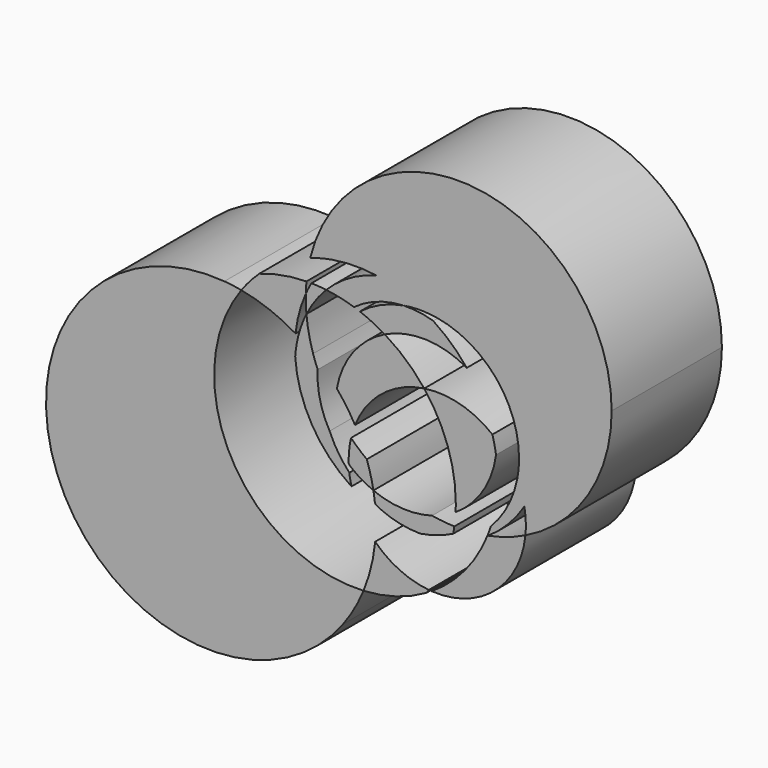
from build123d import *

# Parameters (mm, degrees)
F1_DEPTH = 25.4


with BuildPart() as f1:
    # F0 (on Front) → F1 (new body)
    with BuildSketch(Plane.XZ):
        with BuildLine():
            ThreePointArc((40.1538575824, -54.5525371766), (34.8112838881, -53.101159825), (30.2607130008, -49.9480828366))
            ThreePointArc((30.2607130008, -49.9480828366), (29.5067805021, -54.3549736685), (28.1146409687, -58.6036262239))
            ThreePointArc((28.1146409687, -58.6036262239), (34.1030907269, -57.5733618162), (39.691420026, -55.1872455363))
            ThreePointArc((39.691420026, -55.1872455363), (39.9249388458, -54.8715671271), (40.1538575824, -54.5525371766))
        make_face()
    extrude(amount=F1_DEPTH)


with BuildPart() as f1b:
    # F0 (on Front) → F1, piece 2 (new body)
    with BuildSketch(Plane.XZ):
        with BuildLine():
            ThreePointArc((24.3295831314, -65.2665911695), (26.4328949575, -62.0548490079), (28.1146409687, -58.6036262239))
            ThreePointArc((28.1146409687, -58.6036262239), (3.7618317001, -44.9945627843), (5.5896871945, -17.1570903547))
            ThreePointArc((5.5896871945, -17.1570903547), (4.0379815695, -16.9081548594), (2.4754848513, -16.7397409859))
            ThreePointArc((2.4754848513, -16.7397409859), (-6.670828805, -50.0432179604), (24.3295831314, -65.2665911695))
        make_face()
        with BuildLine():
            ThreePointArc((2.4754848513, -16.7397409859), (-27.7189775168, -59.5222653089), (24.3295831314, -65.2665911695))
            ThreePointArc((24.3295831314, -65.2665911695), (-6.670828805, -50.0432179604), (2.4754848513, -16.7397409859))
        make_face()
    extrude(amount=F1_DEPTH)


with BuildPart() as f1c:
    # F0 (on Front) → F1, piece 3 (new body)
    with BuildSketch(Plane.XZ):
        with BuildLine():
            ThreePointArc((15.5259313509, -24.7108479388), (18.6165177504, -34.7842088044), (25.8966178224, -42.4015880363))
            ThreePointArc((25.8966178224, -42.4015880363), (25.6616341127, -41.3572292778), (25.4955819125, -40.2997184139))
            ThreePointArc((25.4955819125, -40.2997184139), (23.4256571039, -37.6786317178), (21.8713846988, -34.7224650322))
            ThreePointArc((21.8713846988, -34.7224650322), (20.0913666116, -30.2566972991), (19.6726895469, -25.4675162258))
            ThreePointArc((19.6726895469, -25.4675162258), (19.221825797, -24.3258278708), (18.8210952423, -23.1655927897))
            ThreePointArc((18.8210952423, -23.1655927897), (17.4751466685, -22.1634611108), (16.075953424, -21.2371222257))
            ThreePointArc((16.075953424, -21.2371222257), (15.7246867633, -22.9619109348), (15.5259313509, -24.7108479388))
        make_face()
        with BuildLine():
            ThreePointArc((17.5902280452, -17.1382927375), (16.7211824063, -19.1463639854), (16.075953424, -21.2371222257))
            ThreePointArc((16.075953424, -21.2371222257), (17.4751466685, -22.1634611108), (18.8210952423, -23.1655927897))
            ThreePointArc((18.8210952423, -23.1655927897), (18.0407428379, -20.1856217155), (17.5902280452, -17.1382927375))
        make_face()
    extrude(amount=F1_DEPTH)


with BuildPart() as f1d:
    # F0 (on Front) → F1, piece 4 (new body)
    with BuildSketch(Plane.XZ):
        with BuildLine():
            ThreePointArc((8.9074729487, -13.4113681026), (7.1586729424, -15.2045936945), (5.5896871945, -17.1570903547))
            ThreePointArc((5.5896871945, -17.1570903547), (10.7582958294, -18.606057575), (15.5914806817, -20.94151158))
            ThreePointArc((15.5914806817, -20.94151158), (16.2501882549, -17.3285688299), (17.4789014653, -13.8677141914))
            ThreePointArc((17.4789014653, -13.8677141914), (17.5218559184, -12.8490388813), (17.6016231545, -11.8325834418))
            ThreePointArc((17.6016231545, -11.8325834418), (13.1897424114, -12.265100016), (8.9074729487, -13.4113681026))
        make_face()
    extrude(amount=F1_DEPTH)


with BuildPart() as f1e:
    # F0 (on Front) → F1, piece 5 (new body)
    with BuildSketch(Plane.XZ):
        with BuildLine():
            ThreePointArc((50.9276188863, -42.3062252748), (46.7662943353, -49.2544379076), (40.6765473403, -54.5938444613))
            ThreePointArc((40.6765473403, -54.5938444613), (52.276756188, -50.7389787125), (57.9506689588, -39.9116268146))
            ThreePointArc((57.9506689588, -39.9116268146), (54.5873270883, -41.2815480667), (51.0757678908, -42.2076715883))
            ThreePointArc((51.0757678908, -42.2076715883), (51.0017892703, -42.257092564), (50.9276188863, -42.3062252748))
        make_face()
    extrude(amount=F1_DEPTH)


with BuildPart() as f1f:
    # F0 (on Front) → F1, piece 6 (new body)
    with BuildSketch(Plane.XZ):
        with BuildLine():
            ThreePointArc((29.9343874447, -41.7375034561), (30.0945281638, -42.7386739982), (30.2211937836, -43.744627936))
            ThreePointArc((30.2211937836, -43.744627936), (30.7074945796, -44.0520833186), (31.204438934, -44.3420205277))
            ThreePointArc((31.204438934, -44.3420205277), (34.8084393601, -45.5256885647), (38.5798125698, -45.9338958727))
            ThreePointArc((38.5798125698, -45.9338958727), (41.6890159042, -45.2005751575), (44.6424357179, -43.9831122014))
            ThreePointArc((44.6424357179, -43.9831122014), (44.7545364965, -43.3536151903), (44.8517491914, -42.721647815))
            ThreePointArc((44.8517491914, -42.721647815), (42.7970382383, -42.5875979854), (40.7575952062, -42.3039105235))
            ThreePointArc((40.7575952062, -42.3039105235), (35.2982122915, -42.9336942044), (29.9343874447, -41.7375034561))
        make_face()
    extrude(amount=F1_DEPTH)


with BuildPart() as f1g:
    # F0 (on Front) → F1, piece 7 (new body)
    with BuildSketch(Plane.XZ):
        with BuildLine():
            ThreePointArc((58.0307088051, -38.2968299091), (58.0106865683, -39.1052195774), (57.9506689588, -39.9116268146))
            ThreePointArc((57.9506689588, -39.9116268146), (69.5436503466, -29.5130224408), (73.8457056162, -14.5457076903))
            ThreePointArc((73.8457056162, -14.5457076903), (49.056653384, 13.4361560453), (18.2902101299, -7.7984331473))
            ThreePointArc((18.2902101299, -7.7984331473), (20.3676668553, -7.1857892567), (22.4887407194, -6.747377754))
            ThreePointArc((22.4887407194, -6.747377754), (47.2916450309, -2.1862580033), (61.2010402451, -23.2223365456))
            ThreePointArc((61.2010402451, -23.2223365456), (60.3220490691, -29.5007146335), (57.7526664727, -35.2963103729))
            ThreePointArc((57.7526664727, -35.2963103729), (57.9610496417, -36.7901427298), (58.0307088051, -38.2968299091))
        make_face()
        with BuildLine():
            ThreePointArc((51.5809438877, -40.5006277219), (51.2847425976, -41.3710254533), (50.9580903246, -42.2304588174))
            ThreePointArc((50.9580903246, -42.2304588174), (51.0169412202, -42.219127754), (51.0757678908, -42.2076715883))
            ThreePointArc((51.0757678908, -42.2076715883), (54.7814604512, -39.1067758035), (57.7526664727, -35.2963103729))
            ThreePointArc((57.7526664727, -35.2963103729), (57.2273138462, -33.2379593231), (56.4391944195, -31.2652271578))
            ThreePointArc((56.4391944195, -31.2652271578), (54.6885472182, -36.2398384797), (51.5809438877, -40.5006277219))
        make_face()
        with BuildLine():
            ThreePointArc((30.4962956225, -6.6797554599), (25.5094366348, -8.7234981349), (21.2464283719, -12.020831487))
            ThreePointArc((21.2464283719, -12.020831487), (23.8314740731, -12.4577169776), (26.3621830346, -13.1424376226))
            ThreePointArc((26.3621830346, -13.1424376226), (30.6712198814, -10.8607569892), (35.458676282, -9.9365674679))
            ThreePointArc((35.458676282, -9.9365674679), (37.4014358799, -9.6982527409), (39.3585631952, -9.6706586179))
            ThreePointArc((39.3585631952, -9.6706586179), (35.0624037675, -7.7752680174), (30.4962956225, -6.6797554599))
        make_face()
        with BuildLine():
            ThreePointArc((61.2010402451, -23.2223365456), (47.2916450309, -2.1862580033), (22.4887407194, -6.747377754))
            ThreePointArc((22.4887407194, -6.747377754), (26.4899111925, -6.4048589093), (30.4962956225, -6.6797554599))
            ThreePointArc((30.4962956225, -6.6797554599), (44.2759524191, -8.0348709228), (53.8971199923, -17.9922005789))
            ThreePointArc((53.8971199923, -17.9922005789), (56.0400887398, -22.6869112297), (56.7742198891, -27.7951080352))
            ThreePointArc((56.7742198891, -27.7951080352), (56.6902692508, -29.538235167), (56.4391944195, -31.2652271578))
            ThreePointArc((56.4391944195, -31.2652271578), (57.2273138462, -33.2379593231), (57.7526664727, -35.2963103729))
            ThreePointArc((57.7526664727, -35.2963103729), (60.3220490691, -29.5007146335), (61.2010402451, -23.2223365456))
        make_face()
        with BuildLine():
            ThreePointArc((53.8971199923, -17.9922005789), (44.2759524191, -8.0348709228), (30.4962956225, -6.6797554599))
            ThreePointArc((30.4962956225, -6.6797554599), (35.0624037675, -7.7752680174), (39.3585631952, -9.6706586179))
            ThreePointArc((39.3585631952, -9.6706586179), (47.6460065242, -12.0525947694), (53.8971199923, -17.9922005789))
        make_face()
    extrude(amount=F1_DEPTH)


with BuildPart() as f1h:
    # F0 (on Front) → F1, piece 8 (new body)
    with BuildSketch(Plane.XZ):
        with BuildLine():
            ThreePointArc((25.6211827252, -39.1560673783), (27.6790096014, -40.6118249025), (29.9343874447, -41.7375034561))
            ThreePointArc((29.9343874447, -41.7375034561), (29.4205430771, -39.3836074861), (28.7219041832, -37.0777961393))
            ThreePointArc((28.7219041832, -37.0777961393), (27.2210036067, -35.8671250202), (25.8063894155, -34.5566694548))
            ThreePointArc((25.8063894155, -34.5566694548), (25.4551400683, -36.6539261554), (25.3794041172, -38.7790439964))
            ThreePointArc((25.3794041172, -38.7790439964), (25.4989862537, -38.9683939513), (25.6211827252, -39.1560673783))
        make_face()
    extrude(amount=F1_DEPTH)


with BuildPart() as f1i:
    # F0 (on Front) → F1, piece 9 (new body)
    with BuildSketch(Plane.XZ):
        with BuildLine():
            ThreePointArc((18.5160606443, -11.8335602694), (17.9720702659, -12.8376809675), (17.4789014653, -13.8677141914))
            ThreePointArc((17.4789014653, -13.8677141914), (17.4870617924, -15.5046204085), (17.5902280452, -17.1382927375))
            ThreePointArc((17.5902280452, -17.1382927375), (19.2165746577, -14.4354180997), (21.2464283719, -12.020831487))
            ThreePointArc((21.2464283719, -12.020831487), (19.8836109137, -11.8926942742), (18.5160606443, -11.8335602694))
        make_face()
    extrude(amount=F1_DEPTH)


with BuildPart() as f1j:
    # F0 (on Front) → F1, piece 10 (new body)
    with BuildSketch(Plane.XZ):
        with BuildLine():
            ThreePointArc((23.1989496039, -27.3925757669), (24.988667911, -29.7260062824), (26.5445537779, -32.221443871))
            ThreePointArc((26.5445537779, -32.221443871), (31.5800674362, -25.4827792883), (39.3017660933, -22.1449105057))
            ThreePointArc((39.3017660933, -22.1449105057), (35.9559801688, -18.608500995), (32.0312678982, -15.7280306735))
            ThreePointArc((32.0312678982, -15.7280306735), (26.218280873, -20.5026341621), (23.1989496039, -27.3925757669))
        make_face()
    extrude(amount=F1_DEPTH)


with BuildPart() as f1k:
    # F0 (on Front) → F1, piece 11 (new body)
    with BuildSketch(Plane.XZ):
        with BuildLine():
            ThreePointArc((45.1199353433, -38.9192253351), (45.1106157855, -39.6297514098), (45.0826635243, -40.3397886117))
            ThreePointArc((45.0826635243, -40.3397886117), (50.1017921487, -35.2983013137), (52.5349959324, -28.6134104641))
            ThreePointArc((52.5349959324, -28.6134104641), (52.2512002854, -27.0582791448), (51.8738445479, -25.5231648048))
            ThreePointArc((51.8738445479, -25.5231648048), (45.9390130106, -22.5270281049), (39.3017660933, -22.1449105057))
            ThreePointArc((39.3017660933, -22.1449105057), (43.6240948292, -30.0418843563), (45.1199353433, -38.9192253351))
        make_face()
    extrude(amount=F1_DEPTH)


with BuildPart() as f1l:
    # F0 (on Front) → F1, piece 12 (new body)
    with BuildSketch(Plane.XZ):
        with BuildLine():
            ThreePointArc((35.458676282, -9.9365674679), (31.2325863434, -11.2355838156), (27.4463006765, -13.5184154981))
            ThreePointArc((27.4463006765, -13.5184154981), (29.7907916271, -14.5153074856), (32.0312678982, -15.7280306735))
            ThreePointArc((32.0312678982, -15.7280306735), (39.651377077, -14.1119977804), (47.1414811046, -16.2511489823))
            ThreePointArc((47.1414811046, -16.2511489823), (44.2775224684, -13.1942630568), (40.9617154104, -10.6345298313))
            ThreePointArc((40.9617154104, -10.6345298313), (38.2397055228, -10.0528815127), (35.458676282, -9.9365674679))
        make_face()
    extrude(amount=F1_DEPTH)


solid = Compound([f1.part, f1b.part, f1c.part, f1d.part, f1e.part, f1f.part, f1g.part, f1h.part, f1i.part, f1j.part, f1k.part, f1l.part])
